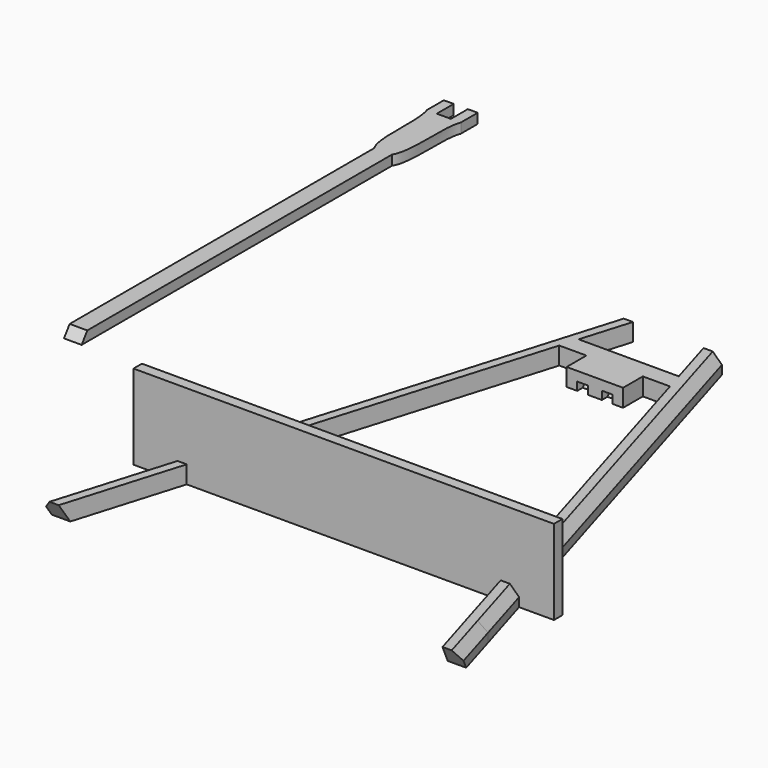
from build123d import *

# Parameters (mm, degrees)
F1_DEPTH     = 5
F3_DEPTH     = 24
F4_W         = 16
F4_H         = 5
F5_DEPTH     = 7
F7_W         = 3
F7_H         = 3
F8_DEPTH     = 5
F9_W         = 2.8
F9_H         = 6
F10_DEPTH    = 2.8
F11_SIZE2    = 1.99999
F11_SIZE     = 2.79999
F13_W        = 140.8556848764
F13_H        = 22.6161023602
F14_DEPTH    = 2
F15_T1_DEPTH = 31.0827660092
F15_T3_DEPTH = 31.0827642559
F17_DEPTH    = 1.6
F18_SIZE     = 2.5


# Not quite as in the source:
# - a fillet or chamfer that OpenCascade refuses, or shapes differently, is made with other operations: its cross-section is extruded or revolved along the edge and cut away or added
# - a fillet or chamfer is up to 0.001 mm smaller than in the source, because OpenCascade refuses the exact size


with BuildPart() as f1:
    # F0 (on Top) → F1 (new body)
    with BuildSketch(Plane.XY):
        Polygon((-11.4133255483, 64.60974645), (-7.2133255483, 78.60974645), (-12.4334788322, 78.60974645), (-52.2133255483, -53.9897426034), (-52.2133255483, -71.39025355), (-41.7133255483, -36.39025355), (-40.8133255483, -33.39025355), (-12.9133255483, 59.60974645), align=None)
        Polygon((16.9866744517, 64.60974645), (-11.4133255483, 64.60974645), (-12.9133255483, 59.60974645), (18.4866744517, 59.60974645), align=None)
        Polygon((18.006829489, 78.60974645), (12.7866744517, 78.60974645), (16.9866744517, 64.60974645), (18.4866744517, 59.60974645), (46.3866744517, -33.39025355), (47.2866744517, -36.39025355), (57.7866744517, -71.39025355), (57.7866744517, -53.989736759), align=None)
        Polygon((46.3866744517, -33.39025355), (-40.8133255483, -33.39025355), (-41.7133255483, -36.39025355), (47.2866744517, -36.39025355), align=None)
        Polygon((-52.2133255483, -71.39025355), (-52.2133255483, -53.9897426034), (-57.0024570015, -69.953514114), align=None)
        Polygon((62.5758075135, -69.9535136315), (57.7866744517, -53.989736759), (57.7866744517, -71.39025355), align=None)
    extrude(amount=F1_DEPTH)

    # F2 (on face) → F3 (join)
    with BuildSketch(Plane(origin=(0, 0, 0), x_dir=(1, 0, 0), z_dir=(0, 0, -1))):
        Polygon((-56.8133255483, 33.39025355), (-40.8133255483, 33.39025355), (46.3866744517, 33.39025355), (62.3866744517, 33.39025355), (62.3866744517, 36.39025355), (47.2866744517, 36.39025355), (-41.7133255483, 36.39025355), (-56.8133255483, 36.39025355), align=None)
    extrude(amount=-F3_DEPTH)

    # F4 (on face) → F5 (join)
    with BuildSketch(Plane.XZ.offset(-59.60974645)):
        with Locations((2.7866744517, 2.5)):
            Rectangle(F4_W, F4_H)
    extrude(amount=F5_DEPTH)

    # F7 (on face) → F8 (cut)
    with BuildSketch(Plane(origin=(0, 21.7370799257, 25.905243094), x_dir=(1, 0, 0), z_dir=(0, 0.6427876097, 0.7660444431))):
        with Locations((6.2866744517, 40.3014039219)):
            Rectangle(F7_W, F7_H)
        with Locations((-0.7133255483, 40.3014039219)):
            Rectangle(F7_W, F7_H)
    extrude(amount=F8_DEPTH, mode=Mode.SUBTRACT)

    # F13 (on 3pt) → F14 (cut)
    with BuildSketch(Plane.XZ.offset(71.39025355)):
        with Locations((4.5045018196, 1.0812641121)):
            Rectangle(F13_W, F13_H)
    extrude(amount=-F14_DEPTH, mode=Mode.SUBTRACT)

    # F15: chamfer of 5 x 3 on 2 edges, made by hand

    # F15_s2 → F15_t1 (cut)
    with BuildSketch(Plane.YZ.offset(44.2553689658)):
        Polygon((-66.39025355, 0), (-69.39025355, 5), (-69.39025355, 0), align=None)
    extrude(amount=F15_T1_DEPTH, mode=Mode.SUBTRACT)

    # F15_s4 → F15_t3 (cut)
    with BuildSketch(Plane.YZ.offset(-69.7647843182)):
        Polygon((-66.39025355, 0), (-69.39025355, 5), (-69.39025355, 0), align=None)
    extrude(amount=F15_T3_DEPTH, mode=Mode.SUBTRACT)

    # F16 (on face) → F17 (cut)
    with BuildSketch(Plane(origin=(0, -33.39025355, 0), x_dir=(-1, 0, 0), z_dir=(0, 1, 0))):
        with BuildLine():
            add(Edge.make_bspline(
                [(9.2133255483, 14), (9.2133255483, 19.1961524227), (-8.7866744517, 16.5980762114), (-26.7866744517, 14), (-8.7866744517, 11.4019237886), (9.2133255483, 8.8038475773), (9.2133255483, 14)],
                knots=[0, 0, 0, 2.0943951024, 2.0943951024, 4.1887902048, 4.1887902048, 6.2831853072, 6.2831853072, 6.2831853072], degree=2, weights=[1, 0.5, 1, 0.5, 1, 0.5, 1]))
        make_face()
    extrude(amount=-F17_DEPTH, mode=Mode.SUBTRACT)

    # F18
    f18_edges = [f1.edges().sort_by_distance(p)[0] for p in [
        (-29.233479, 22.609746, 5),
        (34.806829, 22.609746, 5),
        (-51.883479, -52.890254, 5),
        (57.456829, -52.890254, 5),
    ]]
    chamfer(f18_edges, length=F18_SIZE)


with BuildPart() as f10:
    # F9 (on Top) → F10 (new body)
    with BuildSketch(Plane.XY):
        with BuildLine():
            Line((-106.6472975697, 1.2893290818), (-101.6472975697, 1.2893290818))
            Line((-101.6472975697, 1.2893290818), (-101.6472975697, 111.2893290818))
            add(Edge.make_bspline(
                [(-101.6472975697, 111.2893290818), (-102.9340378828, 109.355815566), (-105.3605572566, 109.355815566), (-106.6472975697, 111.2893290818)],
                knots=[0.403038575, 0.403038575, 0.403038575, 0.403038575, 0.596961425, 0.596961425, 0.596961425, 0.596961425], degree=3))
            Line((-106.6472975697, 111.2893290818), (-106.6472975697, 1.2893290818))
        make_face()
        with BuildLine():
            Line((-106.6472975697, 111.2893290818), (-101.6472975697, 111.2893290818))
            add(Edge.make_bspline(
                [(-99.3472975697, 132.7641010284), (-101.2220129553, 127.6781910253), (-98.973007346, 115.3078371211), (-101.6472975697, 111.2893290818)],
                knots=[0, 0, 0, 0, 0.403038575, 0.403038575, 0.403038575, 0.403038575], degree=3))
            Line((-99.3472975697, 132.7641010284), (-102.1472975697, 132.7641010284))
            Line((-102.1472975697, 132.7641010284), (-106.1472975697, 132.7641010284))
            Line((-106.1472975697, 132.7641010284), (-108.9472975697, 132.7641010284))
            add(Edge.make_bspline(
                [(-106.6472975697, 111.2893290818), (-109.3215877933, 115.3078371211), (-107.072582184, 127.6781910253), (-108.9472975697, 132.7641010284)],
                knots=[0.596961425, 0.596961425, 0.596961425, 0.596961425, 1, 1, 1, 1], degree=3))
        make_face()
        with Locations((-100.7472975697, 135.7641010284)):
            Rectangle(F9_W, F9_H)
        with Locations((-107.5472975697, 135.7641010284)):
            Rectangle(F9_W, F9_H)
        with BuildLine():
            add(Edge.make_bspline(
                [(-101.6472975697, 111.2893290818), (-102.9340378828, 109.355815566), (-105.3605572566, 109.355815566), (-106.6472975697, 111.2893290818)],
                knots=[0.403038575, 0.403038575, 0.403038575, 0.403038575, 0.596961425, 0.596961425, 0.596961425, 0.596961425], degree=3))
            Line((-101.6472975697, 111.2893290818), (-106.6472975697, 111.2893290818))
        make_face()
    extrude(amount=F10_DEPTH)

    # F11 (size 2.8 and 2 in the source; OpenCascade refuses exactly that, so slightly less here)
    f11_edges = [f10.edges().sort_by_distance(p)[0] for p in [
        (-104.147298, 1.289329, 2.8),
    ]]
    f11_side = f10.faces().sort_by_distance((-104.147298, 1.289329, 1.4))[0]
    chamfer(f11_edges, length=F11_SIZE, length2=F11_SIZE2, reference=f11_side)


solid = Compound([f1.part, f10.part])
